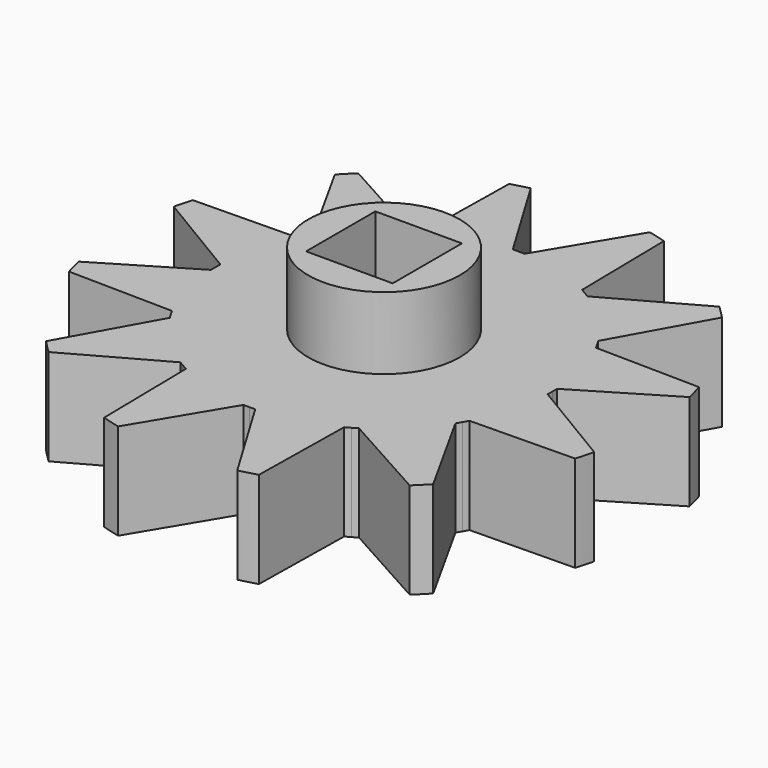
from build123d import *

# Parameters (mm, degrees)
F0_R            = 11
F1_DEPTH        = 4
F3_DEPTH        = 4.001
F3_COPIES_COUNT = 12
F5_R            = 3.15
F6_DEPTH        = 3
F7_W            = 3.6
F7_H            = 3.6
F8_DEPTH        = 7


# Not quite as in the source:
# - a pattern or mirror of a feature is missing from the dataset's text; its kind, count and spacing are read off the source's solid


with BuildPart() as f1:
    # F0 (on Top) → F1 (new body)
    with BuildSketch(Plane.XY):
        Circle(F0_R)
    extrude(amount=F1_DEPTH)

    # F2 (on face) → F3 (cut, through all)
    with BuildSketch(Plane.XY.offset(4)):
        with BuildLine():
            ThreePointArc((-0.2442964769, 6.9957357891), (-0.1221668451, 6.9989338661), (0, 7))
            Line((0, 7), (0, 11))
            ThreePointArc((0, 11), (-1.2452353514, 10.9292904124), (-2.4744615978, 10.7180707126))
            Line((-2.4744615978, 10.7180707126), (-0.2442964769, 6.9957357891))
        make_face()
        with BuildLine():
            Line((0, 11), (0, 7))
            ThreePointArc((0, 7), (0.1221668451, 6.9989338661), (0.2442964769, 6.9957357891))
            Line((0.2442964769, 6.9957357891), (2.4744615978, 10.7180707126))
            ThreePointArc((2.4744615978, 10.7180707126), (1.2452353514, 10.9292904124), (0, 11))
        make_face()
    f3 = extrude(amount=-F3_DEPTH, mode=Mode.SUBTRACT)

    # F3_copies: F3 ×12 about axis
    f3_copies_axis = Axis((0, 0, 0), (0, 0, 1))
    for i in range(1, F3_COPIES_COUNT):
        add(f3.rotate(f3_copies_axis, i * 360 / F3_COPIES_COUNT), mode=Mode.SUBTRACT)

    # F5 (on face) → F6 (join)
    with BuildSketch(Plane.XY.offset(4)):
        Circle(F5_R)
    extrude(amount=F6_DEPTH)

    # F7 (on face) → F8 (cut, through all)
    with BuildSketch(Plane.XY.offset(7)):
        Rectangle(F7_W, F7_H)
    extrude(amount=-F8_DEPTH, mode=Mode.SUBTRACT)


solid = f1.part
